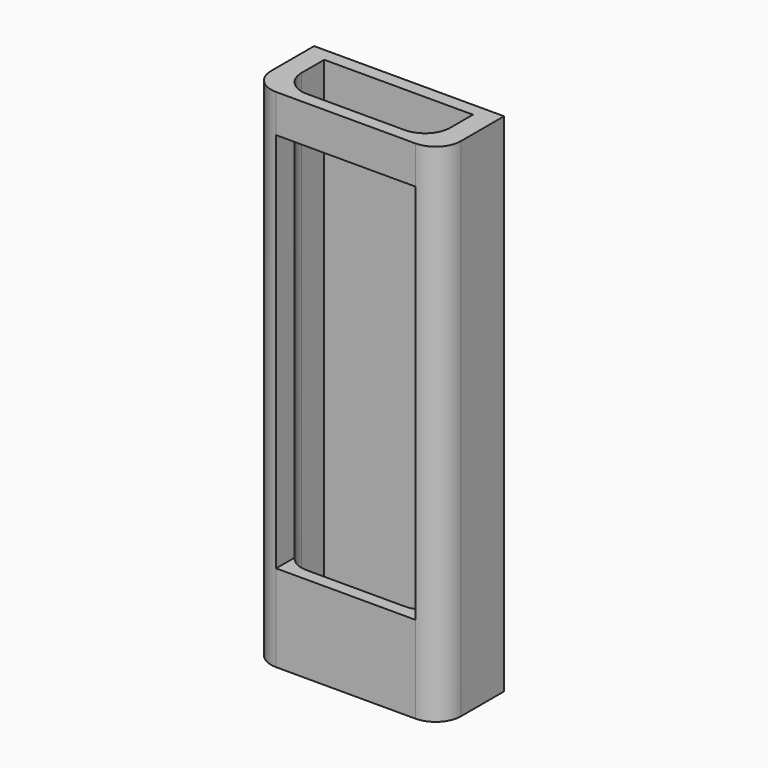
from build123d import *

# Parameters (mm, degrees)
F0_W         = 38.1
F0_H         = 101.6
F1_DEPTH     = 15.875
F2_W         = 27.94
F2_H         = 76.5175
F3_DEPTH     = 12.7
F4_W         = 29.8249544576
F4_H         = 10.7437949628
F5_DEPTH     = 100.23084
F6_T4_DEPTH  = 100.23084
F6_T10_DEPTH = 100.23084
F6_T16_DEPTH = 100.23084
F6_T23_DEPTH = 100.23084
F6_T29_DEPTH = 100.23084
F6_T35_DEPTH = 100.23084
F6_T41_DEPTH = 100.23084
F6_T47_DEPTH = 100.23084
F6_T54_DEPTH = 100.23084
F6_T60_DEPTH = 100.23084
F6_T63_DEPTH = 127


# Not quite as in the source:
# - a fillet or chamfer that OpenCascade refuses, or shapes differently, is made with other operations: its cross-section is extruded or revolved along the edge and cut away or added


with BuildPart() as f1:
    # F0 (on Front) → F1 (new body)
    with BuildSketch(Plane.XZ):
        with Locations((-29.7519958138, -32.7344046354)):
            Rectangle(F0_W, F0_H)
    extrude(amount=F1_DEPTH)

    # F2 (on face) → F3 (cut)
    with BuildSketch(Plane.XZ.offset(15.875)):
        with Locations((-29.7519958138, -27.8131546354)):
            Rectangle(F2_W, F2_H)
    extrude(amount=-F3_DEPTH, mode=Mode.SUBTRACT)

    # F4 (on face) → F5 (cut)
    with BuildSketch(Plane.XY.offset(18.0655953646)):
        with Locations((-29.750072863, -8.0031603575)):
            Rectangle(F4_W, F4_H)
    extrude(amount=-F5_DEPTH, mode=Mode.SUBTRACT)

    # F6: fillet of radius 5.08 on 4 edges, made by hand


with BuildPart() as f6_tool2:
    # F6_s3 → F6_t4 (new body)
    with BuildSketch(Plane.XY.offset(18.0655953646)):
        with BuildLine():
            ThreePointArc((-19.9175956342, -13.3750578389), (-16.3254931857, -11.8871602873), (-14.8375956342, -8.2950578389))
            Line((-14.8375956342, -8.2950578389), (-14.8375956342, -13.3750578389))
            Line((-14.8375956342, -13.3750578389), (-19.9175956342, -13.3750578389))
        make_face()
    extrude(amount=-F6_T4_DEPTH)

    split(bisect_by=Plane.YZ.offset(-15.7819958138), keep=Keep.BOTTOM)

    split(bisect_by=Plane.XY.offset(10.4455953646), keep=Keep.TOP)


with BuildPart() as f1_1:
    add(f1.part)

    # F6_t1: union F6_tool2
    add(f6_tool2.part)


with BuildPart() as f6_tool8:
    # F6_s9 → F6_t10 (new body)
    with BuildSketch(Plane.XY.offset(18.0655953646)):
        with BuildLine():
            ThreePointArc((-19.9175956342, -13.3750578389), (-16.3254931857, -11.8871602873), (-14.8375956342, -8.2950578389))
            Line((-14.8375956342, -8.2950578389), (-14.8375956342, -13.3750578389))
            Line((-14.8375956342, -13.3750578389), (-19.9175956342, -13.3750578389))
        make_face()
    extrude(amount=-F6_T10_DEPTH)

    split(bisect_by=Plane.YZ.offset(-15.7819958138), keep=Keep.TOP)

    split(bisect_by=Plane.XY.offset(10.4455953646), keep=Keep.TOP)


with BuildPart() as f1_2:
    add(f1_1.part)

    # F6_t7: union F6_tool8
    add(f6_tool8.part)


with BuildPart() as f6_tool14:
    # F6_s15 → F6_t16 (new body)
    with BuildSketch(Plane.XY.offset(18.0655953646)):
        with BuildLine():
            ThreePointArc((-19.9175956342, -13.3750578389), (-16.3254931857, -11.8871602873), (-14.8375956342, -8.2950578389))
            Line((-14.8375956342, -8.2950578389), (-14.8375956342, -13.3750578389))
            Line((-14.8375956342, -13.3750578389), (-19.9175956342, -13.3750578389))
        make_face()
    extrude(amount=-F6_T16_DEPTH)

    split(bisect_by=Plane.XY.offset(-66.0719046354), keep=Keep.TOP)

    split(bisect_by=Plane.YZ.offset(-15.7819958138), keep=Keep.TOP)

    split(bisect_by=Plane.XY.offset(10.4455953646), keep=Keep.BOTTOM)


with BuildPart() as f1_3:
    add(f1_2.part)

    # F6_t13: union F6_tool14
    add(f6_tool14.part)


with BuildPart() as f6_tool21:
    # F6_s22 → F6_t23 (new body)
    with BuildSketch(Plane.XY.offset(18.0655953646)):
        with BuildLine():
            ThreePointArc((-19.9175956342, -13.3750578389), (-16.3254931857, -11.8871602873), (-14.8375956342, -8.2950578389))
            Line((-14.8375956342, -8.2950578389), (-14.8375956342, -13.3750578389))
            Line((-14.8375956342, -13.3750578389), (-19.9175956342, -13.3750578389))
        make_face()
    extrude(amount=-F6_T23_DEPTH)

    split(bisect_by=Plane.XY.offset(-66.0719046354), keep=Keep.BOTTOM)

    split(bisect_by=Plane.YZ.offset(-15.7819958138), keep=Keep.BOTTOM)


with BuildPart() as f1_4:
    add(f1_3.part)

    # F6_t20: union F6_tool21
    add(f6_tool21.part)


with BuildPart() as f6_tool27:
    # F6_s28 → F6_t29 (new body)
    with BuildSketch(Plane.XY.offset(18.0655953646)):
        with BuildLine():
            ThreePointArc((-19.9175956342, -13.3750578389), (-16.3254931857, -11.8871602873), (-14.8375956342, -8.2950578389))
            Line((-14.8375956342, -8.2950578389), (-14.8375956342, -13.3750578389))
            Line((-14.8375956342, -13.3750578389), (-19.9175956342, -13.3750578389))
        make_face()
    extrude(amount=-F6_T29_DEPTH)

    split(bisect_by=Plane.XY.offset(-66.0719046354), keep=Keep.BOTTOM)

    split(bisect_by=Plane.YZ.offset(-15.7819958138), keep=Keep.TOP)


with BuildPart() as f1_5:
    add(f1_4.part)

    # F6_t26: union F6_tool27
    add(f6_tool27.part)


with BuildPart() as f6_tool33:
    # F6_s34 → F6_t35 (new body)
    with BuildSketch(Plane.XY.offset(18.0655953646)):
        with BuildLine():
            ThreePointArc((-39.5825500917, -13.3750578389), (-43.1746525402, -11.8871602873), (-44.6625500917, -8.2950578389))
            Line((-44.6625500917, -8.2950578389), (-44.6625500917, -13.3750578389))
            Line((-44.6625500917, -13.3750578389), (-39.5825500917, -13.3750578389))
        make_face()
    extrude(amount=-F6_T35_DEPTH)

    split(bisect_by=Plane.YZ.offset(-43.7219958138), keep=Keep.TOP)

    split(bisect_by=Plane.XY.offset(10.4455953646), keep=Keep.TOP)


with BuildPart() as f1_6:
    add(f1_5.part)

    # F6_t32: union F6_tool33
    add(f6_tool33.part)


with BuildPart() as f6_tool39:
    # F6_s40 → F6_t41 (new body)
    with BuildSketch(Plane.XY.offset(18.0655953646)):
        with BuildLine():
            ThreePointArc((-39.5825500917, -13.3750578389), (-43.1746525402, -11.8871602873), (-44.6625500917, -8.2950578389))
            Line((-44.6625500917, -8.2950578389), (-44.6625500917, -13.3750578389))
            Line((-44.6625500917, -13.3750578389), (-39.5825500917, -13.3750578389))
        make_face()
    extrude(amount=-F6_T41_DEPTH)

    split(bisect_by=Plane.YZ.offset(-43.7219958138), keep=Keep.BOTTOM)

    split(bisect_by=Plane.XY.offset(10.4455953646), keep=Keep.TOP)


with BuildPart() as f1_7:
    add(f1_6.part)

    # F6_t38: union F6_tool39
    add(f6_tool39.part)


with BuildPart() as f6_tool45:
    # F6_s46 → F6_t47 (new body)
    with BuildSketch(Plane.XY.offset(18.0655953646)):
        with BuildLine():
            ThreePointArc((-39.5825500917, -13.3750578389), (-43.1746525402, -11.8871602873), (-44.6625500917, -8.2950578389))
            Line((-44.6625500917, -8.2950578389), (-44.6625500917, -13.3750578389))
            Line((-44.6625500917, -13.3750578389), (-39.5825500917, -13.3750578389))
        make_face()
    extrude(amount=-F6_T47_DEPTH)

    split(bisect_by=Plane.YZ.offset(-43.7219958138), keep=Keep.BOTTOM)

    split(bisect_by=Plane.XY.offset(-66.0719046354), keep=Keep.TOP)

    split(bisect_by=Plane.XY.offset(10.4455953646), keep=Keep.BOTTOM)


with BuildPart() as f1_8:
    add(f1_7.part)

    # F6_t44: union F6_tool45
    add(f6_tool45.part)


with BuildPart() as f6_tool52:
    # F6_s53 → F6_t54 (new body)
    with BuildSketch(Plane.XY.offset(18.0655953646)):
        with BuildLine():
            ThreePointArc((-39.5825500917, -13.3750578389), (-43.1746525402, -11.8871602873), (-44.6625500917, -8.2950578389))
            Line((-44.6625500917, -8.2950578389), (-44.6625500917, -13.3750578389))
            Line((-44.6625500917, -13.3750578389), (-39.5825500917, -13.3750578389))
        make_face()
    extrude(amount=-F6_T54_DEPTH)

    split(bisect_by=Plane.YZ.offset(-43.7219958138), keep=Keep.TOP)

    split(bisect_by=Plane.XY.offset(-66.0719046354), keep=Keep.BOTTOM)


with BuildPart() as f1_9:
    add(f1_8.part)

    # F6_t51: union F6_tool52
    add(f6_tool52.part)


with BuildPart() as f6_tool58:
    # F6_s59 → F6_t60 (new body)
    with BuildSketch(Plane.XY.offset(18.0655953646)):
        with BuildLine():
            ThreePointArc((-39.5825500917, -13.3750578389), (-43.1746525402, -11.8871602873), (-44.6625500917, -8.2950578389))
            Line((-44.6625500917, -8.2950578389), (-44.6625500917, -13.3750578389))
            Line((-44.6625500917, -13.3750578389), (-39.5825500917, -13.3750578389))
        make_face()
    extrude(amount=-F6_T60_DEPTH)

    split(bisect_by=Plane.YZ.offset(-43.7219958138), keep=Keep.BOTTOM)

    split(bisect_by=Plane.XY.offset(-66.0719046354), keep=Keep.BOTTOM)


with BuildPart() as f1_10:
    add(f1_9.part)

    # F6_t57: union F6_tool58
    add(f6_tool58.part)

    # F6_s64 → F6_t63 (cut)
    with BuildSketch(Plane.XY.offset(-96.2344046354)):
        with BuildLine():
            ThreePointArc((-10.7019958138, -10.795), (-12.1898933654, -14.3871024484), (-15.7819958138, -15.875))
            Line((-15.7819958138, -15.875), (-10.7019958138, -15.875))
            Line((-10.7019958138, -15.875), (-10.7019958138, -10.795))
        make_face()
        with BuildLine():
            ThreePointArc((-43.7219958138, -15.875), (-47.3140982623, -14.3871024484), (-48.8019958138, -10.795))
            Line((-48.8019958138, -10.795), (-48.8019958138, -15.875))
            Line((-48.8019958138, -15.875), (-43.7219958138, -15.875))
        make_face()
    extrude(amount=F6_T63_DEPTH, mode=Mode.SUBTRACT)


solid = f1_10.part
